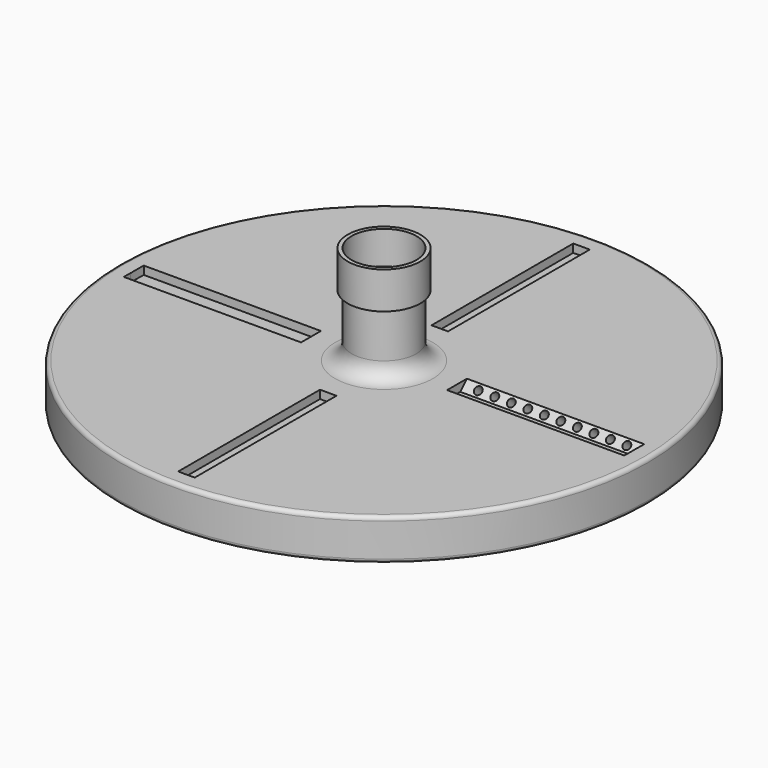
from build123d import *

# Parameters (mm, degrees)
F2_W     = 68.1342573444
F2_H     = 6.35
F3_DEPTH = 3.175
F5_DEPTH = 68.2
F7_DEPTH = 9
F9_DEPTH = 68.2


# Not quite as in the source:
# - a feature names something its author has since deleted; it is built from what else it names


with BuildPart() as f1:
    # F0 (on Front) → F1 (revolve)
    with BuildSketch(Plane.XZ):
        with BuildLine():
            Line((0, -53.9913885295), (0, -50.8))
            Line((0, -50.8), (-96.905, -50.8))
            ThreePointArc((-96.905, -50.8), (-97.9798023074, -50.3548023074), (-98.425, -49.28))
            Line((-98.425, -49.28), (-98.425, -45.97))
            ThreePointArc((-98.425, -45.97), (-97.9798023074, -44.8951976926), (-96.905, -44.45))
            Line((-96.905, -44.45), (-12.47220483, -44.45))
            ThreePointArc((-12.47220483, -44.45), (-11.3974025226, -44.0048023074), (-10.95220483, -42.93))
            Line((-10.95220483, -42.93), (-10.95220483, -39.62))
            Line((-10.95220483, -39.62), (-10.95220483, -38.1))
            Line((-10.95220483, -38.1), (-10.95220483, -36.58))
            Line((-10.95220483, -36.58), (-10.95220483, -12.7))
            Line((-10.95220483, -12.7), (-12.47220483, -12.7))
            Line((-12.47220483, -12.7), (-12.47220483, 0))
            Line((-12.47220483, 0), (-13.99220483, 0))
            Line((-13.99220483, 0), (-13.99220483, -12.7))
            Line((-13.99220483, -12.7), (-13.99220483, -14.22))
            Line((-13.99220483, -14.22), (-12.47220483, -14.22))
            Line((-12.47220483, -14.22), (-12.47220483, -31.75))
            ThreePointArc((-12.47220483, -31.75), (-14.3320767694, -36.2401280605), (-18.82220483, -38.1))
            Line((-18.82220483, -38.1), (-100.08, -38.1))
            ThreePointArc((-100.08, -38.1), (-101.1548023074, -38.5451976926), (-101.6, -39.62))
            Line((-101.6, -39.62), (-101.6, -52.4729063229))
            ThreePointArc((-101.6, -52.4729063229), (-101.1785498226, -53.5234244272), (-100.1479101482, -53.9913885295))
            Line((-100.1479101482, -53.9913885295), (0, -53.9913885295))
        make_face()
    revolve(axis=Axis((0, 0, 8.357311599), (0, 0, 1)))

    # F2 (on face) → F3 (cut)
    with BuildSketch(Plane.XY.offset(-38.1)):
        with BuildLine():
            Line((26.8126719109, -3.175), (94.9469292552, -3.175))
            ThreePointArc((94.9469292552, -3.175), (95, 0), (94.9469292552, 3.175))
            Line((94.9469292552, 3.175), (26.8126719109, 3.175))
            Line((26.8126719109, 3.175), (26.8126719109, -3.175))
        make_face()
        with BuildLine():
            Line((3.175, -94.9469292552), (3.175, -26.8126719109))
            Line((3.175, -26.8126719109), (-3.175, -26.8126719109))
            Line((-3.175, -26.8126719109), (-3.175, -94.9469292552))
            ThreePointArc((-3.175, -94.9469292552), (0, -95), (3.175, -94.9469292552))
        make_face()
        with Locations((-60.8798005831, 0)):
            Rectangle(F2_W, F2_H)
        with BuildLine():
            Line((-94.9469292552, -3.175), (-94.9469292552, 3.175))
            ThreePointArc((-94.9469292552, 3.175), (-95, 0), (-94.9469292552, -3.175))
        make_face()
        with BuildLine():
            Line((3.175, 26.8126719109), (3.175, 94.9469292552))
            ThreePointArc((3.175, 94.9469292552), (0, 95), (-3.175, 94.9469292552))
            Line((-3.175, 94.9469292552), (-3.175, 26.8126719109))
            Line((-3.175, 26.8126719109), (3.175, 26.8126719109))
        make_face()
    extrude(amount=-F3_DEPTH, mode=Mode.SUBTRACT)

    # F4 (on face) → F5 (cut)
    with BuildSketch(Plane(origin=(-26.8126719109, 0, 0), x_dir=(0, -1, 0), z_dir=(-1, 0, 0))):
        Polygon((6.35, -38.1), (3.175, -38.1), (3.175, -41.275), align=None)
    extrude(amount=F5_DEPTH, mode=Mode.SUBTRACT)

    # F6 (on face) → F7 (cut)
    with BuildSketch(Plane(origin=(0, 22.225, -22.225), x_dir=(1, 0, 0), z_dir=(0, -0.7071067812, 0.7071067812))):
        with BuildLine():
            Line((30.9640646577, -24.6957043329), (32.4640646577, -24.6957043329))
            Line((32.4640646577, -24.6957043329), (33.9640646577, -24.6957043329))
            ThreePointArc((33.9640646577, -24.6957043329), (32.4640646577, -23.1957043329), (30.9640646577, -24.6957043329))
        make_face()
        with BuildLine():
            Line((33.9640646577, -24.6957043329), (32.4640646577, -24.6957043329))
            Line((32.4640646577, -24.6957043329), (30.9640646577, -24.6957043329))
            ThreePointArc((30.9640646577, -24.6957043329), (32.4640646577, -26.1957043329), (33.9640646577, -24.6957043329))
        make_face()
        with BuildLine():
            ThreePointArc((91.1140646577, -24.6957043329), (89.6140646577, -23.1957043329), (88.1140646577, -24.6957043329))
            Line((88.1140646577, -24.6957043329), (89.6140646577, -24.6957043329))
            Line((89.6140646577, -24.6957043329), (91.1140646577, -24.6957043329))
        make_face()
        with BuildLine():
            Line((89.6140646577, -24.6957043329), (88.1140646577, -24.6957043329))
            ThreePointArc((88.1140646577, -24.6957043329), (89.6140646577, -26.1957043329), (91.1140646577, -24.6957043329))
            Line((91.1140646577, -24.6957043329), (89.6140646577, -24.6957043329))
        make_face()
        with BuildLine():
            ThreePointArc((84.7640646577, -24.6957043329), (83.2640646577, -23.1957043329), (81.7640646577, -24.6957043329))
            Line((81.7640646577, -24.6957043329), (83.2640646577, -24.6957043329))
            Line((83.2640646577, -24.6957043329), (84.7640646577, -24.6957043329))
        make_face()
        with BuildLine():
            Line((83.2640646577, -24.6957043329), (81.7640646577, -24.6957043329))
            ThreePointArc((81.7640646577, -24.6957043329), (83.2640646577, -26.1957043329), (84.7640646577, -24.6957043329))
            Line((84.7640646577, -24.6957043329), (83.2640646577, -24.6957043329))
        make_face()
        with BuildLine():
            ThreePointArc((78.4140646577, -24.6957043329), (76.9140646577, -23.1957043329), (75.4140646577, -24.6957043329))
            Line((75.4140646577, -24.6957043329), (76.9140646577, -24.6957043329))
            Line((76.9140646577, -24.6957043329), (78.4140646577, -24.6957043329))
        make_face()
        with BuildLine():
            Line((76.9140646577, -24.6957043329), (75.4140646577, -24.6957043329))
            ThreePointArc((75.4140646577, -24.6957043329), (76.9140646577, -26.1957043329), (78.4140646577, -24.6957043329))
            Line((78.4140646577, -24.6957043329), (76.9140646577, -24.6957043329))
        make_face()
        with BuildLine():
            ThreePointArc((72.0640646577, -24.6957043329), (70.5640646577, -23.1957043329), (69.0640646577, -24.6957043329))
            Line((69.0640646577, -24.6957043329), (70.5640646577, -24.6957043329))
            Line((70.5640646577, -24.6957043329), (72.0640646577, -24.6957043329))
        make_face()
        with BuildLine():
            Line((70.5640646577, -24.6957043329), (69.0640646577, -24.6957043329))
            ThreePointArc((69.0640646577, -24.6957043329), (70.5640646577, -26.1957043329), (72.0640646577, -24.6957043329))
            Line((72.0640646577, -24.6957043329), (70.5640646577, -24.6957043329))
        make_face()
        with BuildLine():
            ThreePointArc((65.7140646577, -24.6957043329), (64.2140646577, -23.1957043329), (62.7140646577, -24.6957043329))
            Line((62.7140646577, -24.6957043329), (64.2140646577, -24.6957043329))
            Line((64.2140646577, -24.6957043329), (65.7140646577, -24.6957043329))
        make_face()
        with BuildLine():
            Line((64.2140646577, -24.6957043329), (62.7140646577, -24.6957043329))
            ThreePointArc((62.7140646577, -24.6957043329), (64.2140646577, -26.1957043329), (65.7140646577, -24.6957043329))
            Line((65.7140646577, -24.6957043329), (64.2140646577, -24.6957043329))
        make_face()
        with BuildLine():
            ThreePointArc((59.3640646577, -24.6957043329), (57.8640646577, -23.1957043329), (56.3640646577, -24.6957043329))
            Line((56.3640646577, -24.6957043329), (57.8640646577, -24.6957043329))
            Line((57.8640646577, -24.6957043329), (59.3640646577, -24.6957043329))
        make_face()
        with BuildLine():
            Line((57.8640646577, -24.6957043329), (56.3640646577, -24.6957043329))
            ThreePointArc((56.3640646577, -24.6957043329), (57.8640646577, -26.1957043329), (59.3640646577, -24.6957043329))
            Line((59.3640646577, -24.6957043329), (57.8640646577, -24.6957043329))
        make_face()
        with BuildLine():
            ThreePointArc((53.0140646577, -24.6957043329), (51.5140646577, -23.1957043329), (50.0140646577, -24.6957043329))
            Line((50.0140646577, -24.6957043329), (51.5140646577, -24.6957043329))
            Line((51.5140646577, -24.6957043329), (53.0140646577, -24.6957043329))
        make_face()
        with BuildLine():
            Line((51.5140646577, -24.6957043329), (50.0140646577, -24.6957043329))
            ThreePointArc((50.0140646577, -24.6957043329), (51.5140646577, -26.1957043329), (53.0140646577, -24.6957043329))
            Line((53.0140646577, -24.6957043329), (51.5140646577, -24.6957043329))
        make_face()
        with BuildLine():
            ThreePointArc((46.6640646577, -24.6957043329), (45.1640646577, -23.1957043329), (43.6640646577, -24.6957043329))
            Line((43.6640646577, -24.6957043329), (45.1640646577, -24.6957043329))
            Line((45.1640646577, -24.6957043329), (46.6640646577, -24.6957043329))
        make_face()
        with BuildLine():
            Line((45.1640646577, -24.6957043329), (43.6640646577, -24.6957043329))
            ThreePointArc((43.6640646577, -24.6957043329), (45.1640646577, -26.1957043329), (46.6640646577, -24.6957043329))
            Line((46.6640646577, -24.6957043329), (45.1640646577, -24.6957043329))
        make_face()
        with BuildLine():
            ThreePointArc((40.3140646577, -24.6957043329), (38.8140646577, -23.1957043329), (37.3140646577, -24.6957043329))
            Line((37.3140646577, -24.6957043329), (38.8140646577, -24.6957043329))
            Line((38.8140646577, -24.6957043329), (40.3140646577, -24.6957043329))
        make_face()
        with BuildLine():
            Line((38.8140646577, -24.6957043329), (37.3140646577, -24.6957043329))
            ThreePointArc((37.3140646577, -24.6957043329), (38.8140646577, -26.1957043329), (40.3140646577, -24.6957043329))
            Line((40.3140646577, -24.6957043329), (38.8140646577, -24.6957043329))
        make_face()
    extrude(amount=-F7_DEPTH, mode=Mode.SUBTRACT)

    # F8 (on face) → F9 (cut)
    with BuildSketch(Plane.YZ.offset(26.8126719109)):
        Polygon((6.35, -38.1), (3.175, -38.1), (3.175, -41.275), align=None)
    extrude(amount=F9_DEPTH, mode=Mode.SUBTRACT)


solid = f1.part
